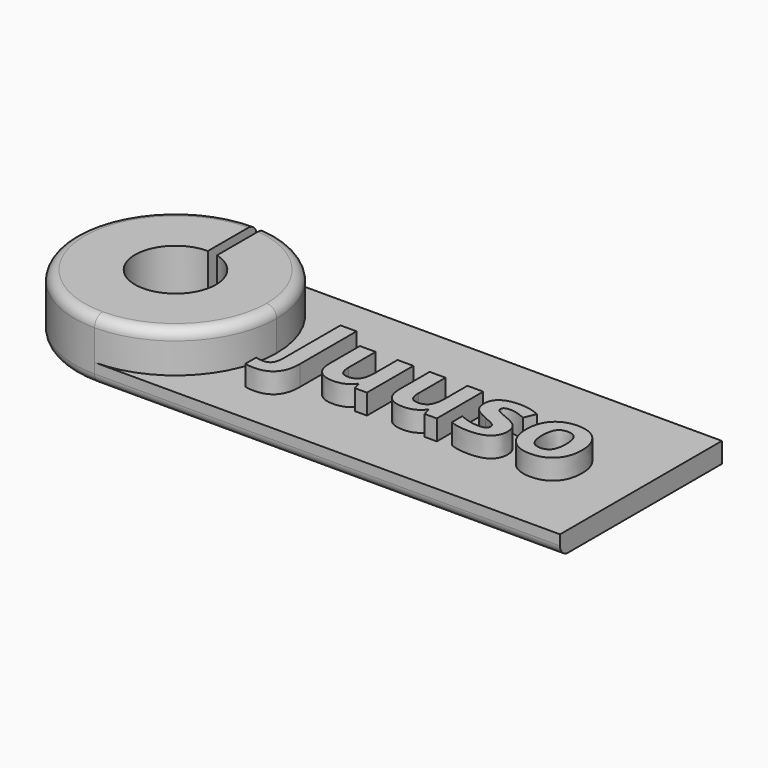
from build123d import *

# Parameters (mm, degrees)
F1_DEPTH     = 3
F2_DEPTH     = 1
F0_TEXT_SIZE = 5.252503146
F3_DEPTH     = 2
F4_R         = 0.5


# Not quite as in the source:
# - Text() gives the source's letters only with a copy of the font that has no kerning and outlines rounded to 1/6400 em; it was checked with that copy


with BuildPart() as f1:
    # F0 (on Top) → F1 (new body)
    with BuildSketch(Plane.XY):
        with BuildLine():
            Line((0, 2), (0, 5))
            ThreePointArc((0, 5), (-5, 0), (0, -5))
            ThreePointArc((0, -5), (3.5355339059, -3.5355339059), (5, 0))
            ThreePointArc((5, 0), (3.7080992435, 3.3541019662), (0.5, 4.9749371855))
            Line((0.5, 4.9749371855), (0.5, 1.9364916731))
            ThreePointArc((0.5, 1.9364916731), (1.5811388301, 1.2247448714), (2, 0))
            ThreePointArc((2, 0), (-1.4142135624, -1.4142135624), (0, 2))
        make_face()
    extrude(amount=F1_DEPTH)

    # F0 (on Top) → F2 (join)
    with BuildSketch(Plane.XY):
        with BuildLine():
            ThreePointArc((5, 0), (3.5355339059, -3.5355339059), (0, -5))
            Line((0, -5), (23, -5))
            Line((23, -5), (23, 5))
            Line((23, 5), (0.5, 5))
            Line((0.5, 5), (0.5, 4.9749371855))
            ThreePointArc((0.5, 4.9749371855), (3.7080992435, 3.3541019662), (5, 0))
        make_face()
        with BuildLine():
            add(Edge.make_bspline(
                [(7.1719076915, -2.665081318), (6.8719405196, -3.0089561334), (6.2843167302, -3.0089561334)],
                knots=[0, 0, 0, 1, 1, 1], degree=2))
            add(Edge.make_bspline(
                [(6.2843167302, -3.0089561334), (6.0151259439, -3.0089561334), (5.8148742615, -2.9523275838)],
                knots=[0, 0, 0, 1, 1, 1], degree=2))
            Line((5.8148742615, -2.9523275838), (5.8148742615, -2.2908404689))
            add(Edge.make_bspline(
                [(5.8148742615, -2.2908404689), (6.0200501656, -2.3417240931), (6.1891151106, -2.3417240931)],
                knots=[0, 0, 0, 1, 1, 1], degree=2))
            add(Edge.make_bspline(
                [(6.1891151106, -2.3417240931), (6.4509195643, -2.3417240931), (6.5637663116, -2.1788144252)],
                knots=[0, 0, 0, 1, 1, 1], degree=2))
            add(Edge.make_bspline(
                [(6.5637663116, -2.1788144252), (6.6766130589, -2.0159047573), (6.6766130589, -1.6695678311)],
                knots=[0, 0, 0, 1, 1, 1], degree=2))
            Line((6.6766130589, -1.6695678311), (6.6766130589, 1.8438643514))
            Line((6.6766130589, 1.8438643514), (7.4718748633, 1.8438643514))
            Line((7.4718748633, 1.8438643514), (7.4718748633, -1.6646436094))
            add(Edge.make_bspline(
                [(7.4718748633, -1.6646436094), (7.4718748633, -2.3212065027), (7.1719076915, -2.665081318)],
                knots=[0, 0, 0, 1, 1, 1], degree=2))
        make_face(mode=Mode.SUBTRACT)
        with BuildLine():
            Line((10.9853070458, -1.9059304727), (10.3853727021, -1.9059304727))
            Line((10.3853727021, -1.9059304727), (10.2803226392, -1.5390759561))
            Line((10.2803226392, -1.5390759561), (10.2392874584, -1.5390759561))
            add(Edge.make_bspline(
                [(10.2392874584, -1.5390759561), (10.1137198051, -1.7393276385), (9.882691737, -1.8484812195)],
                knots=[0, 0, 0, 1, 1, 1], degree=2))
            add(Edge.make_bspline(
                [(9.882691737, -1.8484812195), (9.6516636689, -1.9576348006), (9.3570310706, -1.9576348006)],
                knots=[0, 0, 0, 1, 1, 1], degree=2))
            add(Edge.make_bspline(
                [(9.3570310706, -1.9576348006), (8.8514776428, -1.9576348006), (8.5950077626, -1.6868026071)],
                knots=[0, 0, 0, 1, 1, 1], degree=2))
            add(Edge.make_bspline(
                [(8.5950077626, -1.6868026071), (8.3385378824, -1.4159704136), (8.3385378824, -0.907954875)],
                knots=[0, 0, 0, 1, 1, 1], degree=2))
            Line((8.3385378824, -0.907954875), (8.3385378824, 0.9616079636))
            Line((8.3385378824, 0.9616079636), (9.120668429, 0.9616079636))
            Line((9.120668429, 0.9616079636), (9.120668429, -0.7134481178))
            add(Edge.make_bspline(
                [(9.120668429, -0.7134481178), (9.120668429, -1.0236740849), (9.2310530654, -1.1787870684)],
                knots=[0, 0, 0, 1, 1, 1], degree=2))
            add(Edge.make_bspline(
                [(9.2310530654, -1.1787870684), (9.3414377019, -1.333900052), (9.5827245651, -1.333900052)],
                knots=[0, 0, 0, 1, 1, 1], degree=2))
            add(Edge.make_bspline(
                [(9.5827245651, -1.333900052), (9.9110060118, -1.333900052), (10.0570912555, -1.1147721863)],
                knots=[0, 0, 0, 1, 1, 1], degree=2))
            add(Edge.make_bspline(
                [(10.0570912555, -1.1147721863), (10.2031764993, -0.8956443207), (10.2031764993, -0.3876287821)],
                knots=[0, 0, 0, 1, 1, 1], degree=2))
            Line((10.2031764993, -0.3876287821), (10.2031764993, 0.9616079636))
            Line((10.2031764993, 0.9616079636), (10.9853070458, 0.9616079636))
            Line((10.9853070458, 0.9616079636), (10.9853070458, -1.9059304727))
        make_face(mode=Mode.SUBTRACT)
        with BuildLine():
            Line((14.4371864571, -1.9059304727), (13.8372521134, -1.9059304727))
            Line((13.8372521134, -1.9059304727), (13.7322020505, -1.5390759561))
            Line((13.7322020505, -1.5390759561), (13.6911668697, -1.5390759561))
            add(Edge.make_bspline(
                [(13.6911668697, -1.5390759561), (13.5655992163, -1.7393276385), (13.3345711483, -1.8484812195)],
                knots=[0, 0, 0, 1, 1, 1], degree=2))
            add(Edge.make_bspline(
                [(13.3345711483, -1.8484812195), (13.1035430802, -1.9576348006), (12.8089104819, -1.9576348006)],
                knots=[0, 0, 0, 1, 1, 1], degree=2))
            add(Edge.make_bspline(
                [(12.8089104819, -1.9576348006), (12.3033570541, -1.9576348006), (12.0468871739, -1.6868026071)],
                knots=[0, 0, 0, 1, 1, 1], degree=2))
            add(Edge.make_bspline(
                [(12.0468871739, -1.6868026071), (11.7904172937, -1.4159704136), (11.7904172937, -0.907954875)],
                knots=[0, 0, 0, 1, 1, 1], degree=2))
            Line((11.7904172937, -0.907954875), (11.7904172937, 0.9616079636))
            Line((11.7904172937, 0.9616079636), (12.5725478403, 0.9616079636))
            Line((12.5725478403, 0.9616079636), (12.5725478403, -0.7134481178))
            add(Edge.make_bspline(
                [(12.5725478403, -0.7134481178), (12.5725478403, -1.0236740849), (12.6829324767, -1.1787870684)],
                knots=[0, 0, 0, 1, 1, 1], degree=2))
            add(Edge.make_bspline(
                [(12.6829324767, -1.1787870684), (12.7933171131, -1.333900052), (13.0346039764, -1.333900052)],
                knots=[0, 0, 0, 1, 1, 1], degree=2))
            add(Edge.make_bspline(
                [(13.0346039764, -1.333900052), (13.362885423, -1.333900052), (13.5089706668, -1.1147721863)],
                knots=[0, 0, 0, 1, 1, 1], degree=2))
            add(Edge.make_bspline(
                [(13.5089706668, -1.1147721863), (13.6550559105, -0.8956443207), (13.6550559105, -0.3876287821)],
                knots=[0, 0, 0, 1, 1, 1], degree=2))
            Line((13.6550559105, -0.3876287821), (13.6550559105, 0.9616079636))
            Line((13.6550559105, 0.9616079636), (14.4371864571, 0.9616079636))
            Line((14.4371864571, 0.9616079636), (14.4371864571, -1.9059304727))
        make_face(mode=Mode.SUBTRACT)
        with BuildLine():
            add(Edge.make_bspline(
                [(17.1840814618, -0.6875959539), (17.2587654909, -0.841477882), (17.2587654909, -1.0540401187)],
                knots=[0, 0, 0, 1, 1, 1], degree=2))
            add(Edge.make_bspline(
                [(17.2587654909, -1.0540401187), (17.2587654909, -1.4955786644), (16.9522326901, -1.7266067325)],
                knots=[0, 0, 0, 1, 1, 1], degree=2))
            add(Edge.make_bspline(
                [(16.9522326901, -1.7266067325), (16.6456998893, -1.9576348006), (16.0350963986, -1.9576348006)],
                knots=[0, 0, 0, 1, 1, 1], degree=2))
            add(Edge.make_bspline(
                [(16.0350963986, -1.9576348006), (15.7224083207, -1.9576348006), (15.5016390478, -1.9149582125)],
                knots=[0, 0, 0, 1, 1, 1], degree=2))
            add(Edge.make_bspline(
                [(15.5016390478, -1.9149582125), (15.280869775, -1.8722816244), (15.0888251287, -1.7902112628)],
                knots=[0, 0, 0, 1, 1, 1], degree=2))
            Line((15.0888251287, -1.7902112628), (15.0888251287, -1.1443175165))
            add(Edge.make_bspline(
                [(15.0888251287, -1.1443175165), (15.3063115871, -1.2469054686), (15.5796058914, -1.3162549242)],
                knots=[0, 0, 0, 1, 1, 1], degree=2))
            add(Edge.make_bspline(
                [(15.5796058914, -1.3162549242), (15.8529001957, -1.3856043798), (16.0605382107, -1.3856043798)],
                knots=[0, 0, 0, 1, 1, 1], degree=2))
            add(Edge.make_bspline(
                [(16.0605382107, -1.3856043798), (16.4864833877, -1.3856043798), (16.4864833877, -1.1393932948)],
                knots=[0, 0, 0, 1, 1, 1], degree=2))
            add(Edge.make_bspline(
                [(16.4864833877, -1.1393932948), (16.4864833877, -1.0466537862), (16.4298548382, -0.9887941812)],
                knots=[0, 0, 0, 1, 1, 1], degree=2))
            add(Edge.make_bspline(
                [(16.4298548382, -0.9887941812), (16.3732262886, -0.9309345762), (16.2349377292, -0.8578919543)],
                knots=[0, 0, 0, 1, 1, 1], degree=2))
            add(Edge.make_bspline(
                [(16.2349377292, -0.8578919543), (16.0966491698, -0.7848493325), (15.8660314536, -0.6880063057)],
                knots=[0, 0, 0, 1, 1, 1], degree=2))
            add(Edge.make_bspline(
                [(15.8660314536, -0.6880063057), (15.5352878961, -0.5493073945), (15.3797645608, -0.4311260737)],
                knots=[0, 0, 0, 1, 1, 1], degree=2))
            add(Edge.make_bspline(
                [(15.3797645608, -0.4311260737), (15.2242412254, -0.3129447529), (15.1540710662, -0.1602938803)],
                knots=[0, 0, 0, 1, 1, 1], degree=2))
            add(Edge.make_bspline(
                [(15.1540710662, -0.1602938803), (15.083900907, -0.0076430076), (15.083900907, 0.2147676725)],
                knots=[0, 0, 0, 1, 1, 1], degree=2))
            add(Edge.make_bspline(
                [(15.083900907, 0.2147676725), (15.083900907, 0.5972155578), (15.3797645608, 0.8060846282)],
                knots=[0, 0, 0, 1, 1, 1], degree=2))
            add(Edge.make_bspline(
                [(15.3797645608, 0.8060846282), (15.6756282145, 1.0149536987), (16.2197547123, 1.0149536987)],
                knots=[0, 0, 0, 1, 1, 1], degree=2))
            add(Edge.make_bspline(
                [(16.2197547123, 1.0149536987), (16.7376186944, 1.0149536987), (17.2275787535, 0.7892602041)],
                knots=[0, 0, 0, 1, 1, 1], degree=2))
            Line((17.2275787535, 0.7892602041), (16.9920368155, 0.2254368195))
            add(Edge.make_bspline(
                [(16.9920368155, 0.2254368195), (16.7761917643, 0.3173556246), (16.5890713398, 0.376446285)],
                knots=[0, 0, 0, 1, 1, 1], degree=2))
            add(Edge.make_bspline(
                [(16.5890713398, 0.376446285), (16.4019509152, 0.4355369454), (16.2066234545, 0.4355369454)],
                knots=[0, 0, 0, 1, 1, 1], degree=2))
            add(Edge.make_bspline(
                [(16.2066234545, 0.4355369454), (15.8602865283, 0.4355369454), (15.8602865283, 0.2484165208)],
                knots=[0, 0, 0, 1, 1, 1], degree=2))
            add(Edge.make_bspline(
                [(15.8602865283, 0.2484165208), (15.8602865283, 0.1433664579), (15.9719022201, 0.0662203179)],
                knots=[0, 0, 0, 1, 1, 1], degree=2))
            add(Edge.make_bspline(
                [(15.9719022201, 0.0662203179), (16.083517912, -0.0109258221), (16.4610415756, -0.1619352875)],
                knots=[0, 0, 0, 1, 1, 1], degree=2))
            add(Edge.make_bspline(
                [(16.4610415756, -0.1619352875), (16.7967093548, -0.2981720879), (16.9530533937, -0.4159430568)],
                knots=[0, 0, 0, 1, 1, 1], degree=2))
            add(Edge.make_bspline(
                [(16.9530533937, -0.4159430568), (17.1093974327, -0.5337140258), (17.1840814618, -0.6875959539)],
                knots=[0, 0, 0, 1, 1, 1], degree=2))
        make_face(mode=Mode.SUBTRACT)
        with BuildLine():
            add(Edge.make_bspline(
                [(20.3052173156, 0.3202280872), (20.4742822606, -0.0158500438), (20.4742822606, -0.4672370329)],
                knots=[0, 0, 0, 1, 1, 1], degree=2))
            add(Edge.make_bspline(
                [(20.4742822606, -0.4672370329), (20.4742822606, -1.1672972178), (20.1049656331, -1.5624660092)],
                knots=[0, 0, 0, 1, 1, 1], degree=2))
            add(Edge.make_bspline(
                [(20.1049656331, -1.5624660092), (19.7356490057, -1.9576348006), (19.0766240016, -1.9576348006)],
                knots=[0, 0, 0, 1, 1, 1], degree=2))
            add(Edge.make_bspline(
                [(19.0766240016, -1.9576348006), (18.6638100825, -1.9576348006), (18.3482495419, -1.7766696531)],
                knots=[0, 0, 0, 1, 1, 1], degree=2))
            add(Edge.make_bspline(
                [(18.3482495419, -1.7766696531), (18.0326890013, -1.5957045056), (17.8636240563, -1.2571642638)],
                knots=[0, 0, 0, 1, 1, 1], degree=2))
            add(Edge.make_bspline(
                [(17.8636240563, -1.2571642638), (17.6945591113, -0.918624022), (17.6945591113, -0.4672370329)],
                knots=[0, 0, 0, 1, 1, 1], degree=2))
            add(Edge.make_bspline(
                [(17.6945591113, -0.4672370329), (17.6945591113, 0.2352852629), (18.0610032761, 0.6251194808)],
                knots=[0, 0, 0, 1, 1, 1], degree=2))
            add(Edge.make_bspline(
                [(18.0610032761, 0.6251194808), (18.4274474409, 1.0149536987), (19.0922173703, 1.0149536987)],
                knots=[0, 0, 0, 1, 1, 1], degree=2))
            add(Edge.make_bspline(
                [(19.0922173703, 1.0149536987), (19.5050312894, 1.0149536987), (19.82059183, 0.8356299584)],
                knots=[0, 0, 0, 1, 1, 1], degree=2))
            add(Edge.make_bspline(
                [(19.82059183, 0.8356299584), (20.1361523706, 0.6563062182), (20.3052173156, 0.3202280872)],
                knots=[0, 0, 0, 1, 1, 1], degree=2))
        make_face(mode=Mode.SUBTRACT)
    extrude(amount=F2_DEPTH)



with BuildPart() as f2:
    # F0 (on Top) → F2, piece 2 (new body)
    with BuildSketch(Plane.XY):
        with BuildLine():
            add(Edge.make_bspline(
                [(18.6301612342, 0.1729117881), (18.491462323, -0.038829745), (18.491462323, -0.4672370329)],
                knots=[0, 0, 0, 1, 1, 1], degree=2))
            add(Edge.make_bspline(
                [(18.491462323, -0.4672370329), (18.491462323, -0.8931822099), (18.6313922896, -1.1110790201)],
                knots=[0, 0, 0, 1, 1, 1], degree=2))
            add(Edge.make_bspline(
                [(18.6313922896, -1.1110790201), (18.7713222562, -1.3289758303), (19.086472445, -1.3289758303)],
                knots=[0, 0, 0, 1, 1, 1], degree=2))
            add(Edge.make_bspline(
                [(19.086472445, -1.3289758303), (19.3999812265, -1.3289758303), (19.5370387305, -1.1123100755)],
                knots=[0, 0, 0, 1, 1, 1], degree=2))
            add(Edge.make_bspline(
                [(19.5370387305, -1.1123100755), (19.6740962344, -0.8956443207), (19.6740962344, -0.4672370329)],
                knots=[0, 0, 0, 1, 1, 1], degree=2))
            add(Edge.make_bspline(
                [(19.6740962344, -0.4672370329), (19.6740962344, -0.0412918559), (19.5358076751, 0.1716807326)],
                knots=[0, 0, 0, 1, 1, 1], degree=2))
            add(Edge.make_bspline(
                [(19.5358076751, 0.1716807326), (19.3975191157, 0.3846533211), (19.0815482233, 0.3846533211)],
                knots=[0, 0, 0, 1, 1, 1], degree=2))
            add(Edge.make_bspline(
                [(19.0815482233, 0.3846533211), (18.7688601454, 0.3846533211), (18.6301612342, 0.1729117881)],
                knots=[0, 0, 0, 1, 1, 1], degree=2))
        make_face()
    extrude(amount=F2_DEPTH)


with BuildPart() as f1_1:
    add(f1.part)

    add(f2.part)  # F3 merges F2
    # F0 (on Top) → F3 (join)
    with BuildSketch(Plane.XY):
        with Locations((6.2047084793, -1.9059304727)):
            Text('Juuso', F0_TEXT_SIZE, font='Open Sans', font_style=FontStyle.BOLD, text_align=(TextAlign.LEFT, TextAlign.BOTTOM))
    extrude(amount=F3_DEPTH)

    # F4
    f4_edges = [f1_1.edges().sort_by_distance(p)[0] for p in [
        (-3.535534, -3.535534, 3),
        (-5, 0, 0),
    ]]
    fillet(f4_edges, radius=F4_R)


solid = f1_1.part
